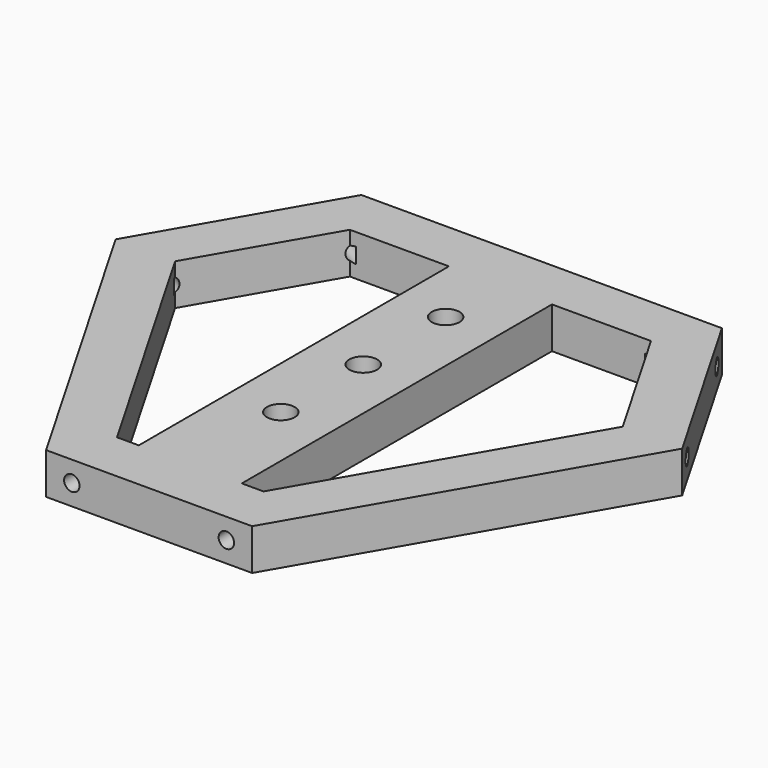
from build123d import *

# Parameters (mm, degrees)
F0_R            = 2.7
F1_DEPTH        = 8
F2_R            = 1.5
F3_DEPTH        = 11
F3_COPIES_COUNT = 3


# Not quite as in the source:
# - a pattern or mirror of a feature is missing from the dataset's text; its kind, count and spacing are read off the source's solid


with BuildPart() as f1:
    # F0 (on Top) → F1 (new body)
    with BuildSketch(Plane.XY):
        Polygon((30.9826352704, 105.0418671526), (-39.0173647296, 105.0418671526), (-59.0173647296, 70.4008510012), (-24.0173647296, 9.7790727363), (15.9826352704, 9.7790727363), (50.9826352704, 70.4008510012), align=None)
        with Locations((-4.0173647296, 41.7405969634)):
            Circle(F0_R, mode=Mode.SUBTRACT)
        Polygon((-14.0173647296, 19.7790727363), (-18.2438620377, 19.7790727363), (-47.4703593458, 70.4008510012), (-33.2438620377, 95.0418671526), (-14.0173647296, 95.0418671526), align=None, mode=Mode.SUBTRACT)
        Polygon((25.2091325785, 95.0418671526), (39.4356298866, 70.4008510012), (10.2091325785, 19.7790727363), (5.9826352704, 19.7790727363), (5.9826352704, 95.0418671526), align=None, mode=Mode.SUBTRACT)
        with Locations((-4.0173647296, 61.7405969634)):
            Circle(F0_R, mode=Mode.SUBTRACT)
        with Locations((-4.0173647296, 81.7405969634)):
            Circle(F0_R, mode=Mode.SUBTRACT)
    extrude(amount=F1_DEPTH)

    # F2 (on face) → F3 (cut)
    with BuildSketch(Plane.XZ.offset(-9.7790727363)):
        with Locations((10.9826352704, 4)):
            Circle(F2_R)
        with Locations((-19.0173647296, 4)):
            Circle(F2_R)
    f3 = extrude(amount=-F3_DEPTH, mode=Mode.SUBTRACT)

    # F3_copies: F3 ×3 about axis
    f3_copies_axis = Axis((-4.017365, 61.740597, 0), (0, 0, 1))
    for i in range(1, F3_COPIES_COUNT):
        add(f3.rotate(f3_copies_axis, i * 360 / F3_COPIES_COUNT), mode=Mode.SUBTRACT)


solid = f1.part
